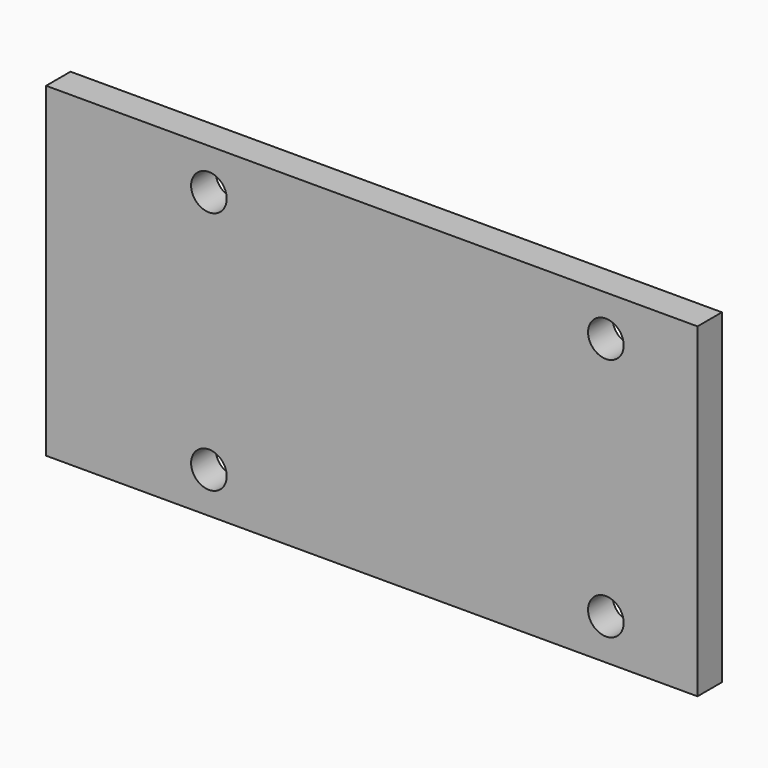
from build123d import *

# Parameters (mm, degrees)
F0_W     = 203.2
F0_H     = 101.6
F1_DEPTH = 9.525
F2_D     = 11.1125
F2_DEPTH = 19.05
F2_TIP   = 3.3385318145


# Not quite as in the source:
# - a length typed as a fraction of an inch, garbled in the dataset ("3 / 203.2 mm" for 3/8 in), is restored


with BuildPart() as f1:
    # F0 (on Front) → F1 (new body)
    with BuildSketch(Plane.XZ):
        with Locations((1.4680749737, 0)):
            Rectangle(F0_W, F0_H)
    extrude(amount=F1_DEPTH)

    # F2
    with Locations(Plane(origin=(0, 0, 0), x_dir=(1, 0, 0), z_dir=(0, 1, 0))):
        with Locations((74.4930749737, -38.1), (-49.3319250263, 38.1), (-49.3319250263, -38.1), (74.4930749737, 38.1)):
            Hole(F2_D / 2, depth=F2_DEPTH)
            with Locations((0, 0, -(F2_DEPTH + F2_TIP / 2))):  # 118° drill point
                Cone(0, F2_D / 2, F2_TIP, mode=Mode.SUBTRACT)


solid = f1.part
